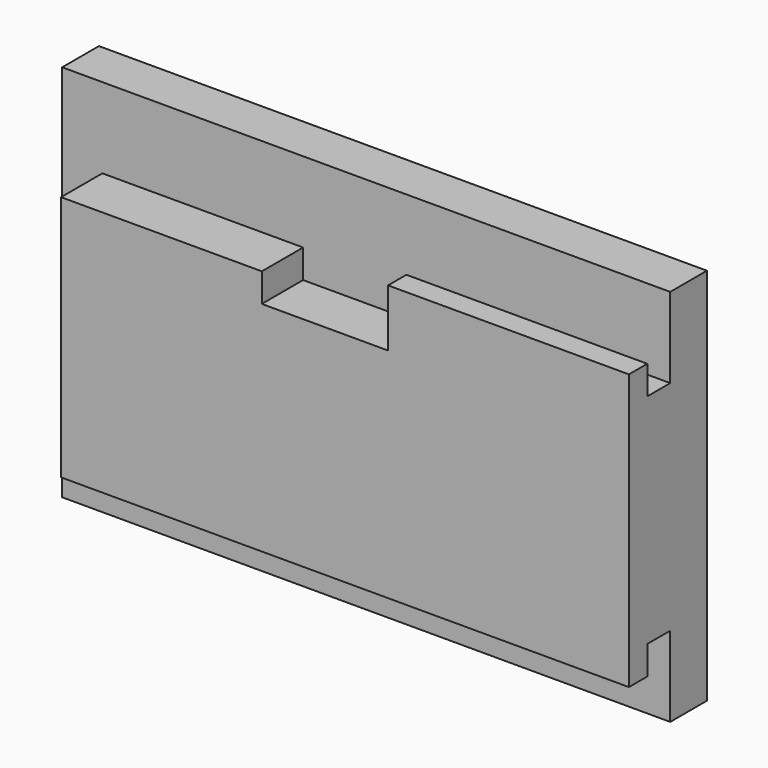
from build123d import *

# Parameters (mm, degrees)
F0_W     = 5.5
F0_H     = 4.5
F0_W_2   = 3.5
F0_H_2   = 2.5
F0_H_3   = 19
F0_W_3   = 11
F1_DEPTH = 4
F0_W_4   = 17.5
F0_W_5   = 46
F2_DEPTH = 8.5
F3_DEPTH = 1
F4_DEPTH = 6.5
F5_DEPTH = 4


with BuildPart() as f1:
    # F0 (on Front) → F1 (new body)
    with BuildSketch(Plane.XZ):
        Polygon((-23, -12), (-26.5, -12), (-26.5, -16.5), (26.5, -16.5), (26.5, -12), (23, -12), align=None)
        with Locations((-2.75, 14.25)):
            Rectangle(F0_W, F0_H)
        with Locations((2.75, 14.25)):
            Rectangle(F0_W, F0_H)
        Polygon((-5.5, 16.5), (-26.5, 16.5), (-26.5, 12), (-23, 12), (-5.5, 12), align=None)
        with Locations((-24.75, 10.75)):
            Rectangle(F0_W_2, F0_H_2)
        with Locations((-24.75, 0)):
            Rectangle(F0_W_2, F0_H_3)
        with Locations((-24.75, -10.75)):
            Rectangle(F0_W_2, F0_H_2)
        Polygon((0, 12), (-5.5, 12), (-5.5, 9.5), (5.5, 9.5), (5.5, 12), align=None)
        with Locations((0, 8.25)):
            Rectangle(F0_W_3, F0_H_2)
        Polygon((26.5, 16.5), (5.5, 16.5), (5.5, 12), (23, 12), (26.5, 12), align=None)
        with Locations((24.75, 10.75)):
            Rectangle(F0_W_2, F0_H_2)
        with Locations((24.75, 0)):
            Rectangle(F0_W_2, F0_H_3)
        with Locations((24.75, -10.75)):
            Rectangle(F0_W_2, F0_H_2)
    extrude(amount=F1_DEPTH)

    # F0 (on Front) → F2 (join)
    with BuildSketch(Plane.XZ):
        Polygon((-5.5, 7), (-5.5, 9.5), (-23, 9.5), (-23, -9.5), (23, -9.5), (23, 9.5), (5.5, 9.5), (5.5, 7), align=None)
        with Locations((14.25, 10.75)):
            Rectangle(F0_W_4, F0_H_2)
        with Locations((0, -10.75)):
            Rectangle(F0_W_5, F0_H_2)
        with Locations((24.75, 10.75)):
            Rectangle(F0_W_2, F0_H_2)
        with Locations((24.75, 0)):
            Rectangle(F0_W_2, F0_H_3)
        with Locations((24.75, -10.75)):
            Rectangle(F0_W_2, F0_H_2)
    extrude(amount=F2_DEPTH)

    # F0 (on Front) → F3 (join)
    with BuildSketch(Plane.XZ):
        with Locations((-2.75, 14.25)):
            Rectangle(F0_W, F0_H)
        with Locations((2.75, 14.25)):
            Rectangle(F0_W, F0_H)
    extrude(amount=F3_DEPTH)

    # F0 (on Front) → F4 (cut)
    with BuildSketch(Plane.XZ):
        with Locations((14.25, 10.75)):
            Rectangle(F0_W_4, F0_H_2)
        with Locations((0, -10.75)):
            Rectangle(F0_W_5, F0_H_2)
        with Locations((24.75, 10.75)):
            Rectangle(F0_W_2, F0_H_2)
        with Locations((24.75, -10.75)):
            Rectangle(F0_W_2, F0_H_2)
    extrude(amount=F4_DEPTH, mode=Mode.SUBTRACT)

    # F0 (on Front) → F5 (join)
    with BuildSketch(Plane.XZ):
        with Locations((14.25, 10.75)):
            Rectangle(F0_W_4, F0_H_2)
        with Locations((-14.25, 10.75)):
            Rectangle(F0_W_4, F0_H_2)
        with Locations((0, -10.75)):
            Rectangle(F0_W_5, F0_H_2)
        with Locations((24.75, 10.75)):
            Rectangle(F0_W_2, F0_H_2)
        with Locations((24.75, -10.75)):
            Rectangle(F0_W_2, F0_H_2)
    extrude(amount=F5_DEPTH)


solid = f1.part
